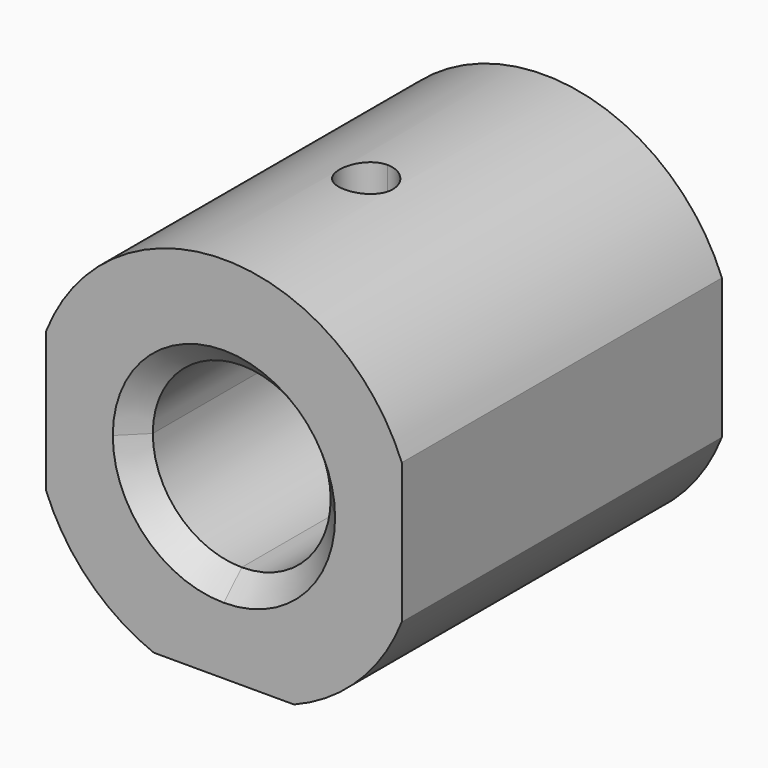
from build123d import *

# Parameters (mm, degrees)
F1_DEPTH = 40
F2_R     = 10
F3_DEPTH = 5
F6_DEPTH = 15
F7_SIZE  = 2.5


with BuildPart() as f1:
    # F0 (on Front) → F1 (new body)
    with BuildSketch(Plane.XZ):
        with BuildLine():
            Line((-20, 0), (-20, -7.889866919))
            ThreePointArc((-20, -7.889866919), (-15.2027957955, -15.2027957955), (-7.889866919, -20))
            Line((-7.889866919, -20), (0, -20))
            Line((0, -20), (0, -10))
            ThreePointArc((0, -10), (-7.0710678119, -7.0710678119), (-10, 0))
            Line((-10, 0), (-20, 0))
        make_face()
        with BuildLine():
            ThreePointArc((7.889866919, -20), (15.2027957955, -15.2027957955), (20, -7.889866919))
            Line((20, -7.889866919), (20, 0))
            Line((20, 0), (10, 0))
            ThreePointArc((10, 0), (7.0710678119, -7.0710678119), (0, -10))
            Line((0, -10), (0, -20))
            Line((0, -20), (7.889866919, -20))
        make_face()
        with BuildLine():
            Line((20, 0), (20, 7.889866919))
            ThreePointArc((20, 7.889866919), (0, 21.5), (-20, 7.889866919))
            Line((-20, 7.889866919), (-20, 0))
            Line((-20, 0), (-10, 0))
            ThreePointArc((-10, 0), (0, 10), (10, 0))
            Line((10, 0), (20, 0))
        make_face()
    extrude(amount=F1_DEPTH)

    # F2 (on face) → F3 (join)
    with BuildSketch(Plane(origin=(0, 0, 0), x_dir=(-1, 0, 0), z_dir=(0, 1, 0))):
        with BuildLine():
            ThreePointArc((20, 7.889866919), (0, 21.5), (-20, 7.889866919))
            Line((-20, 7.889866919), (-20, -7.889866919))
            ThreePointArc((-20, -7.889866919), (-15.2027957955, -15.2027957955), (-7.889866919, -20))
            Line((-7.889866919, -20), (7.889866919, -20))
            ThreePointArc((7.889866919, -20), (15.2027957955, -15.2027957955), (20, -7.889866919))
            Line((20, -7.889866919), (20, 7.889866919))
        make_face()
        Circle(F2_R, mode=Mode.SUBTRACT)
        Circle(F2_R)
    extrude(amount=F3_DEPTH)

    # F5 (on offset) → F6 (cut)
    with BuildSketch(Plane.XY.offset(21.5)):
        with BuildLine():
            ThreePointArc((0, -17), (-2.1213203436, -22.1213203436), (3, -20))
            ThreePointArc((3, -20), (2.1213203436, -17.8786796564), (0, -17))
        make_face()
    extrude(amount=-F6_DEPTH, mode=Mode.SUBTRACT)

    # F7
    f7_edges = [f1.edges().sort_by_distance(p)[0] for p in [
        (10, -40, 0),
    ]]
    chamfer(f7_edges, length=F7_SIZE)


solid = f1.part
